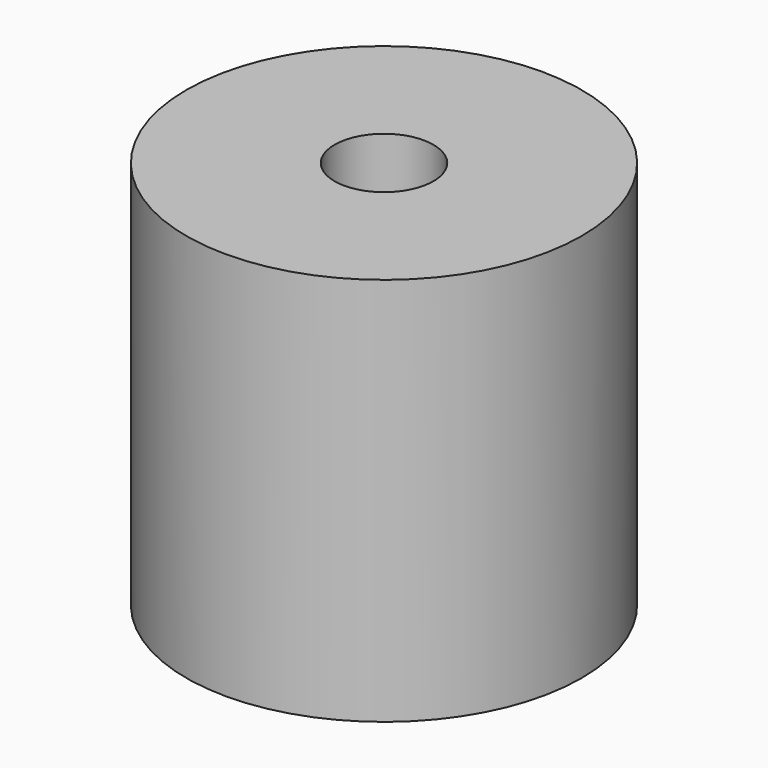
from build123d import *

# Parameters (mm, degrees)
F0_R     = 25.4
F1_DEPTH = 50
F3_D     = 12.7


# Not quite as in the source:
# - a length typed as a fraction of an inch, garbled in the dataset ("3 / 203.2 mm" for 3/8 in), is restored


with BuildPart() as f1:
    # F0 (on Top) → F1 (new body)
    with BuildSketch(Plane.XY):
        Circle(F0_R)
    extrude(amount=F1_DEPTH)

    # F3 (through all)
    with Locations(Plane.XY.offset(50)):
        with Locations((0, 0)):
            Hole(F3_D / 2)


solid = f1.part
